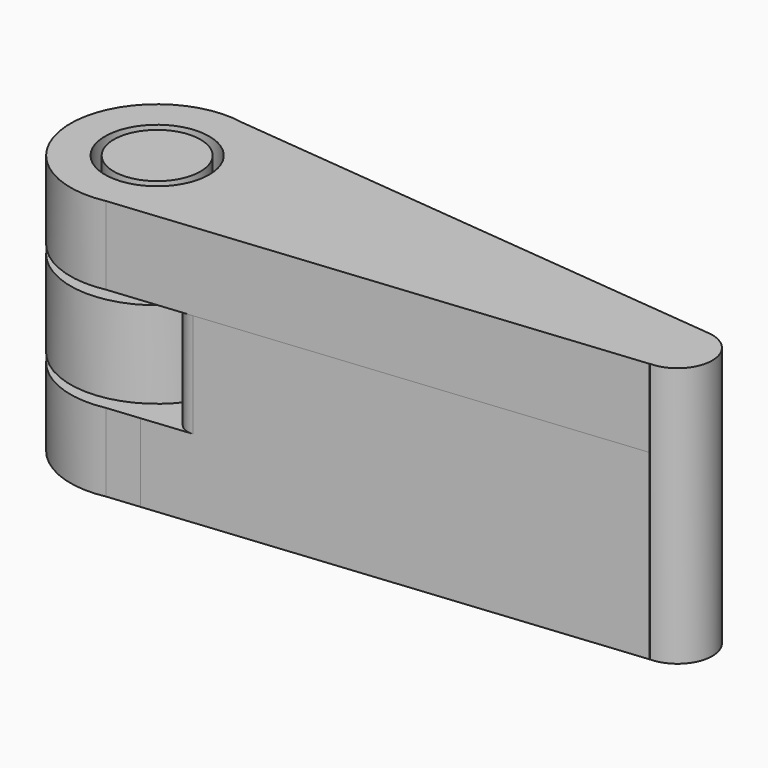
from build123d import *

# Parameters (mm, degrees)
F0_R         = 2.5
F1_DEPTH     = 1.25
F2_R         = 1.25
F3_DEPTH     = 2.5
F4_R         = 1.25
F5_DEPTH     = 2.5
F7_R         = 2.5
F7_R_2       = 1.5
F8_DEPTH     = 2.25
F10_R        = 2.5
F10_R_2      = 1.5
F11_DEPTH    = 2.25
F13_DEPTH    = 2.25
F15_DEPTH    = 3
F16_R        = 1.5
F17_DEPTH    = 2.25
F18_T1_DEPTH = 3


# Not quite as in the source:
# - a fillet or chamfer that OpenCascade refuses, or shapes differently, is made with other operations: its cross-section is extruded or revolved along the edge and cut away or added


with BuildPart() as f1:
    # F0 (on Top) → F1 (new body, symmetric)
    with BuildSketch(Plane.XY):
        Circle(F0_R)
    extrude(amount=F1_DEPTH, both=True)

    # F2 (on face) → F3 (join)
    with BuildSketch(Plane.XY.offset(1.25)):
        Circle(F2_R)
    extrude(amount=F3_DEPTH)

    # F4 (on face) → F5 (join)
    with BuildSketch(Plane(origin=(0, 0, -1.25), x_dir=(1, 0, 0), z_dir=(0, 0, -1))):
        Circle(F4_R)
    extrude(amount=F5_DEPTH)


with BuildPart() as f8:
    # F7 (on offset) → F8 (new body)
    with BuildSketch(Plane.XY.offset(1.5)):
        Circle(F7_R)
        Circle(F7_R_2, mode=Mode.SUBTRACT)
    extrude(amount=F8_DEPTH)

    # F12 (on face) → F13 (join, through all)
    with BuildSketch(Plane.XY.offset(3.75)):
        with BuildLine():
            ThreePointArc((15, -1), (14, 0), (15, 1))
            Line((15, 1), (15, 1.0049547481))
            Line((15, 1.0049547481), (0.4934464972, 2.4508183438))
            ThreePointArc((0.4934464972, 2.4508183438), (1.9343753828, 1.5837272109), (2.5, 0))
            ThreePointArc((2.5, 0), (1.9343753828, -1.5837272109), (0.4934464972, -2.4508183438))
            Line((0.4934464972, -2.4508183438), (15, -1.0049547481))
            Line((15, -1.0049547481), (15, -1))
        make_face()
        with BuildLine():
            ThreePointArc((2.5, 0), (1.9343753828, 1.5837272109), (0.4934464972, 2.4508183438))
            Line((0.4934464972, 2.4508183438), (0, 2.5))
            Line((0, 2.5), (0, 1.5))
            ThreePointArc((0, 1.5), (1.0606601718, 1.0606601718), (1.5, 0))
            ThreePointArc((1.5, 0), (1.0606601718, -1.0606601718), (0, -1.5))
            Line((0, -1.5), (0, -2.5))
            Line((0, -2.5), (0.4934464972, -2.4508183438))
            ThreePointArc((0.4934464972, -2.4508183438), (1.9343753828, -1.5837272109), (2.5, 0))
        make_face()
        with BuildLine():
            Line((0, 1.5), (0, 2.5))
            ThreePointArc((0, 2.5), (-2.5, 0), (0, -2.5))
            Line((0, -2.5), (0, -1.5))
            ThreePointArc((0, -1.5), (-1.5, 0), (0, 1.5))
        make_face()
        with BuildLine():
            ThreePointArc((15, -1), (15.7071067812, -0.7071067812), (16, 0))
            ThreePointArc((16, 0), (15.7071067812, 0.7071067812), (15, 1))
            Line((15, 1), (15, -1))
        make_face()
        with BuildLine():
            Line((15, -1), (15, 1))
            ThreePointArc((15, 1), (14, 0), (15, -1))
        make_face()
    extrude(amount=-F13_DEPTH)

    # F14 (on face) → F15 (join, through all)
    with BuildSketch(Plane(origin=(0, 0, 1.5), x_dir=(1, 0, 0), z_dir=(0, 0, -1))):
        with BuildLine():
            Line((15, 1), (15, 1.0049547481))
            Line((15, 1.0049547481), (1.4131117673, 2.3591555975))
            ThreePointArc((1.4131117673, 2.3591555975), (2.75, 0), (1.4131117673, -2.3591555975))
            Line((1.4131117673, -2.3591555975), (15, -1.0049547481))
            Line((15, -1.0049547481), (15, -1))
            ThreePointArc((15, -1), (16, 0), (15, 1))
        make_face()
    extrude(amount=F15_DEPTH)



with BuildPart() as f11:
    # F10 (on offset) → F11 (new body)
    with BuildSketch(Plane(origin=(0, 0, -1.5), x_dir=(1, 0, 0), z_dir=(0, 0, -1))):
        Circle(F10_R)
        Circle(F10_R_2, mode=Mode.SUBTRACT)
    extrude(amount=F11_DEPTH)


with BuildPart() as f8_1:
    add(f8.part)

    add(f11.part)  # F17 merges F11
    # F16 (on face) → F17 (join, through all)
    with BuildSketch(Plane(origin=(0, 0, -3.75), x_dir=(1, 0, 0), z_dir=(0, 0, -1))):
        with BuildLine():
            Line((0.4934464972, -2.4508183438), (1.4131117673, -2.3591555975))
            ThreePointArc((1.4131117673, -2.3591555975), (2.75, 0), (1.4131117673, 2.3591555975))
            Line((1.4131117673, 2.3591555975), (0.4934464972, 2.4508183438))
            ThreePointArc((0.4934464972, 2.4508183438), (1.9343753828, 1.5837272109), (2.5, 0))
            ThreePointArc((2.5, 0), (1.9343753828, -1.5837272109), (0.4934464972, -2.4508183438))
        make_face()
        with BuildLine():
            Line((0, -2.5), (0.4934464972, -2.4508183438))
            ThreePointArc((0.4934464972, -2.4508183438), (1.9343753828, -1.5837272109), (2.5, 0))
            ThreePointArc((2.5, 0), (1.9343753828, 1.5837272109), (0.4934464972, 2.4508183438))
            Line((0.4934464972, 2.4508183438), (0, 2.5))
            ThreePointArc((0, 2.5), (-2.5, 0), (0, -2.5))
        make_face()
        Circle(F16_R, mode=Mode.SUBTRACT)
        with BuildLine():
            Line((15, -1.0049547481), (15, -1))
            ThreePointArc((15, -1), (16, 0), (15, 1))
            Line((15, 1), (15, 1.0049547481))
            Line((15, 1.0049547481), (1.4131117673, 2.3591555975))
            ThreePointArc((1.4131117673, 2.3591555975), (2.75, 0), (1.4131117673, -2.3591555975))
            Line((1.4131117673, -2.3591555975), (15, -1.0049547481))
        make_face()
    extrude(amount=-F17_DEPTH)

    # F18: fillet of radius 0.5 on 2 edges, made by hand

    # F18_s2 → F18_t1 (cut)
    with BuildSketch(Plane.XY.offset(-1.5)):
        with BuildLine():
            ThreePointArc((2.3318052613, 1.4578011604), (2.331005251, 1.986626711), (2.8053589943, 2.2203907571))
            Line((2.8053589943, 2.2203907571), (1.4131117673, 2.3591555975))
            ThreePointArc((1.4131117673, 2.3591555975), (1.9259311626, 1.9629796629), (2.3318052613, 1.4578011604))
        make_face()
        with BuildLine():
            ThreePointArc((2.8053589943, -2.2203907571), (2.331005251, -1.986626711), (2.3318052613, -1.4578011604))
            ThreePointArc((2.3318052613, -1.4578011604), (1.9259311626, -1.9629796629), (1.4131117673, -2.3591555975))
            Line((1.4131117673, -2.3591555975), (2.8053589943, -2.2203907571))
        make_face()
    extrude(amount=F18_T1_DEPTH, mode=Mode.SUBTRACT)


solid = Compound([f1.part, f8_1.part])
